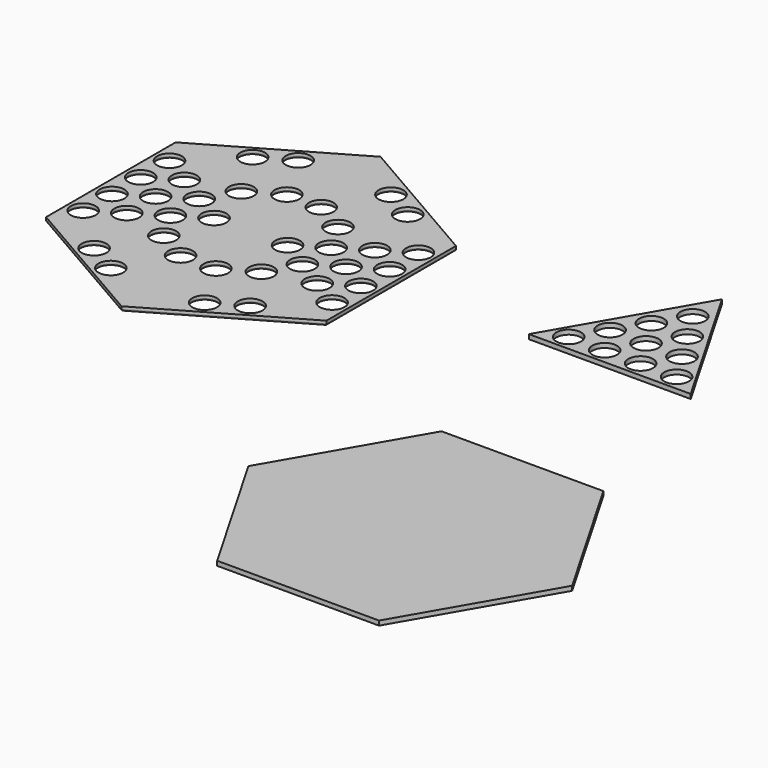
from build123d import *

# Parameters (mm, degrees)
F0_R        = 34.925
F1_DEPTH    = 12.7
F3_DEPTH    = 12.7
F4_T1_DEPTH = 482.6
F4_T3_DEPTH = 482.6
F4_T5_DEPTH = 482.6
F4_T7_DEPTH = 482.6
F4_T9_DEPTH = 482.6


# Not quite as in the source:
# - a fillet or chamfer that OpenCascade refuses, or shapes differently, is made with other operations: its cross-section is extruded or revolved along the edge and cut away or added


with BuildPart() as f1:
    # F0 (on Top) → F1 (new body)
    with BuildSketch(Plane.XY):
        Polygon((784.5862163544, 0), (1241.7862163544, 0), (1013.1862163544, 395.9468146102), align=None)
        with BuildLine():
            ThreePointArc((896.5008747508, 44.45), (870.615129901, 10.7150405169), (831.3299375236, 26.9875))
            ThreePointArc((831.3299375236, 26.9875), (852.5366196006, 78.1849594831), (896.5008747508, 44.45))
        make_face(mode=Mode.SUBTRACT)
        with Locations((963.1758747508, 44.45)):
            Circle(F0_R, mode=Mode.SUBTRACT)
        with Locations((1064.7758747508, 44.45)):
            Circle(F0_R, mode=Mode.SUBTRACT)
        with BuildLine():
            ThreePointArc((1201.3008747508, 44.45), (1200.0064823043, 35.0299224745), (1196.2192506657, 26.3080999065))
            ThreePointArc((1196.2192506657, 26.3080999065), (1132.7452671974, 53.8700775255), (1201.3008747508, 44.45))
        make_face(mode=Mode.SUBTRACT)
        with Locations((912.3758747508, 127)):
            Circle(F0_R, mode=Mode.SUBTRACT)
        with Locations((1013.9758747508, 127)):
            Circle(F0_R, mode=Mode.SUBTRACT)
        with BuildLine():
            ThreePointArc((963.1758747508, 174.625), (938.4801704179, 234.2457043329), (998.1008747508, 209.55))
            ThreePointArc((998.1008747508, 209.55), (987.8715790837, 184.8542956671), (963.1758747508, 174.625))
        make_face(mode=Mode.SUBTRACT)
        with Locations((1115.5758747508, 127)):
            Circle(F0_R, mode=Mode.SUBTRACT)
        with Locations((1064.7758747508, 209.55)):
            Circle(F0_R, mode=Mode.SUBTRACT)
        with BuildLine():
            ThreePointArc((1013.9758747508, 257.175), (989.2801704179, 316.7957043329), (1048.9008747508, 292.1))
            ThreePointArc((1048.9008747508, 292.1), (1038.6715790837, 267.4042956671), (1013.9758747508, 257.175))
        make_face(mode=Mode.SUBTRACT)
    extrude(amount=F1_DEPTH)


with BuildPart() as f1b:
    # F0 (on Top) → F1, piece 2 (new body)
    with BuildSketch(Plane.XY):
        Polygon((0, 0), (0, -457.2), (395.9468146102, -228.6), align=None)
        with Locations((132.4381810245, -329.4103416036)):
            Circle(F0_R, mode=Mode.SUBTRACT)
        with Locations((220.426362049, -278.6103416036)):
            Circle(F0_R, mode=Mode.SUBTRACT)
        with Locations((49.8881810245, -186.4295474388)):
            Circle(F0_R, mode=Mode.SUBTRACT)
        with Locations((137.876362049, -135.6295474388)):
            Circle(F0_R, mode=Mode.SUBTRACT)
        Polygon((-395.9468146102, -228.6), (0, -457.2), (0, 0), align=None)
        with Locations((-220.426362049, -278.6103416036)):
            Circle(F0_R, mode=Mode.SUBTRACT)
        with Locations((-132.4381810245, -329.4103416036)):
            Circle(F0_R, mode=Mode.SUBTRACT)
        with Locations((-49.8881810245, -186.4295474388)):
            Circle(F0_R, mode=Mode.SUBTRACT)
        with Locations((-137.876362049, -135.6295474388)):
            Circle(F0_R, mode=Mode.SUBTRACT)
        Polygon((-395.9468146102, 228.6), (-395.9468146102, -228.6), (0, 0), align=None)
        with Locations((-351.4968146102, -153.1896583964)):
            Circle(F0_R, mode=Mode.SUBTRACT)
        with Locations((-268.9468146102, -102.3896583964)):
            Circle(F0_R, mode=Mode.SUBTRACT)
        with Locations((-351.4968146102, -51.5896583964)):
            Circle(F0_R, mode=Mode.SUBTRACT)
        with Locations((-268.9468146102, -0.7896583964)):
            Circle(F0_R, mode=Mode.SUBTRACT)
        with Locations((-186.3968146102, -51.5896583964)):
            Circle(F0_R, mode=Mode.SUBTRACT)
        with Locations((-103.8468146102, -0.7896583964)):
            Circle(F0_R, mode=Mode.SUBTRACT)
        with Locations((-351.4968146102, 50.0103416036)):
            Circle(F0_R, mode=Mode.SUBTRACT)
        with Locations((-268.9468146102, 100.8103416036)):
            Circle(F0_R, mode=Mode.SUBTRACT)
        with Locations((-186.3968146102, 50.0103416036)):
            Circle(F0_R, mode=Mode.SUBTRACT)
        with Locations((-351.4968146102, 151.6103416036)):
            Circle(F0_R, mode=Mode.SUBTRACT)
        Polygon((0, 0), (395.9468146102, -228.6), (395.9468146102, 228.6), align=None)
        with Locations((351.4968146102, -153.1896583964)):
            Circle(F0_R, mode=Mode.SUBTRACT)
        with Locations((103.8468146102, -0.7896583964)):
            Circle(F0_R, mode=Mode.SUBTRACT)
        with Locations((186.3968146102, -51.5896583964)):
            Circle(F0_R, mode=Mode.SUBTRACT)
        with Locations((268.9468146102, -102.3896583964)):
            Circle(F0_R, mode=Mode.SUBTRACT)
        with Locations((268.9468146102, -0.7896583964)):
            Circle(F0_R, mode=Mode.SUBTRACT)
        with Locations((351.4968146102, -51.5896583964)):
            Circle(F0_R, mode=Mode.SUBTRACT)
        with Locations((186.3968146102, 50.0103416036)):
            Circle(F0_R, mode=Mode.SUBTRACT)
        with Locations((351.4968146102, 50.0103416036)):
            Circle(F0_R, mode=Mode.SUBTRACT)
        with Locations((268.9468146102, 100.8103416036)):
            Circle(F0_R, mode=Mode.SUBTRACT)
        with Locations((351.4968146102, 151.6103416036)):
            Circle(F0_R, mode=Mode.SUBTRACT)
        Polygon((0, 457.2), (0, 0), (395.9468146102, 228.6), align=None)
        with Locations((136.5086335857, 136.4192058352)):
            Circle(F0_R, mode=Mode.SUBTRACT)
        with Locations((48.5204525612, 187.2192058352)):
            Circle(F0_R, mode=Mode.SUBTRACT)
        with Locations((131.0704525612, 330.2)):
            Circle(F0_R, mode=Mode.SUBTRACT)
        with Locations((219.0586335857, 279.4)):
            Circle(F0_R, mode=Mode.SUBTRACT)
        Polygon((-395.9468146102, 228.6), (0, 0), (0, 457.2), align=None)
        with Locations((-136.5086335857, 136.4192058352)):
            Circle(F0_R, mode=Mode.SUBTRACT)
        with Locations((-48.5204525612, 187.2192058352)):
            Circle(F0_R, mode=Mode.SUBTRACT)
        with Locations((-219.0586335857, 279.4)):
            Circle(F0_R, mode=Mode.SUBTRACT)
        with Locations((-131.0704525612, 330.2)):
            Circle(F0_R, mode=Mode.SUBTRACT)
    extrude(amount=F1_DEPTH)

    # F4: fillet of radius 5.08 on 42 edges, made by hand

    # F4_s2 → F4_t1 (cut)
    with BuildSketch(Plane.XZ.offset(-241.3)):
        with BuildLine():
            ThreePointArc((-395.9468146102, 5.08), (-394.4589170587, 1.4878975516), (-390.8668146102, 0))
            Line((-390.8668146102, 0), (-395.9468146102, 0))
            Line((-395.9468146102, 0), (-395.9468146102, 5.08))
        make_face()
        with BuildLine():
            ThreePointArc((395.9468146102, 5.08), (394.4589170587, 1.4878975516), (390.8668146102, 0))
            Line((390.8668146102, 0), (395.9468146102, 0))
            Line((395.9468146102, 0), (395.9468146102, 5.08))
        make_face()
    extrude(amount=F4_T1_DEPTH, mode=Mode.SUBTRACT)

    # F4_s4 → F4_t3 (cut)
    with BuildSketch(Plane(origin=(-208.9719299332, 120.65, 0), x_dir=(0, 0, 1), z_dir=(0.8660254038, -0.5, 0))):
        with BuildLine():
            ThreePointArc((5.08, 395.9468146102), (1.4878975516, 394.4589170587), (0, 390.8668146102))
            Line((0, 390.8668146102), (0, 395.9468146102))
            Line((0, 395.9468146102), (5.08, 395.9468146102))
        make_face()
    extrude(amount=F4_T3_DEPTH, mode=Mode.SUBTRACT)

    # F4_s6 → F4_t5 (cut)
    with BuildSketch(Plane(origin=(-208.9719299332, -120.65, 0), x_dir=(0, 0, 1), z_dir=(0.8660254038, 0.5, 0))):
        with BuildLine():
            ThreePointArc((5.08, 395.9468146102), (1.4878975516, 394.4589170587), (0, 390.8668146102))
            Line((0, 390.8668146102), (0, 395.9468146102))
            Line((0, 395.9468146102), (5.08, 395.9468146102))
        make_face()
    extrude(amount=F4_T5_DEPTH, mode=Mode.SUBTRACT)

    # F4_s8 → F4_t7 (cut)
    with BuildSketch(Plane(origin=(208.9719299332, -120.65, 0), x_dir=(0, 0, 1), z_dir=(-0.8660254038, 0.5, 0))):
        with BuildLine():
            ThreePointArc((5.08, 395.9468146102), (1.4878975516, 394.4589170587), (0, 390.8668146102))
            Line((0, 390.8668146102), (0, 395.9468146102))
            Line((0, 395.9468146102), (5.08, 395.9468146102))
        make_face()
    extrude(amount=F4_T7_DEPTH, mode=Mode.SUBTRACT)

    # F4_s10 → F4_t9 (cut)
    with BuildSketch(Plane(origin=(208.9719299332, 120.65, 0), x_dir=(0, 0, 1), z_dir=(-0.8660254038, -0.5, 0))):
        with BuildLine():
            ThreePointArc((5.08, 395.9468146102), (1.4878975516, 394.4589170587), (0, 390.8668146102))
            Line((0, 390.8668146102), (0, 395.9468146102))
            Line((0, 395.9468146102), (5.08, 395.9468146102))
        make_face()
    extrude(amount=F4_T9_DEPTH, mode=Mode.SUBTRACT)

    # F4_s11 → F4_t12 (revolve, cut)
    with BuildSketch(Plane.XZ.offset(329.4103416036)):
        with BuildLine():
            ThreePointArc((167.3631810245, 5.08), (168.8510785761, 1.4878975516), (172.4431810245, 0))
            Line((172.4431810245, 0), (167.3631810245, 0))
            Line((167.3631810245, 0), (167.3631810245, 5.08))
        make_face()
    revolve(axis=Axis((132.4381810245, -329.4103416036, 0), (0, 0, 1)), mode=Mode.SUBTRACT)

    # F4_s13 → F4_t14 (revolve, cut)
    with BuildSketch(Plane.XZ.offset(278.6103416036)):
        with BuildLine():
            ThreePointArc((255.351362049, 5.08), (256.8392596006, 1.4878975516), (260.431362049, 0))
            Line((260.431362049, 0), (255.351362049, 0))
            Line((255.351362049, 0), (255.351362049, 5.08))
        make_face()
    revolve(axis=Axis((220.426362049, -278.6103416036, 0), (0, 0, 1)), mode=Mode.SUBTRACT)

    # F4_s15 → F4_t16 (revolve, cut)
    with BuildSketch(Plane.XZ.offset(186.4295474388)):
        with BuildLine():
            ThreePointArc((84.8131810245, 5.08), (86.3010785761, 1.4878975516), (89.8931810245, 0))
            Line((89.8931810245, 0), (84.8131810245, 0))
            Line((84.8131810245, 0), (84.8131810245, 5.08))
        make_face()
    revolve(axis=Axis((49.8881810245, -186.4295474388, 0), (0, 0, 1)), mode=Mode.SUBTRACT)

    # F4_s17 → F4_t18 (revolve, cut)
    with BuildSketch(Plane.XZ.offset(135.6295474388)):
        with BuildLine():
            ThreePointArc((172.801362049, 5.08), (174.2892596006, 1.4878975516), (177.881362049, 0))
            Line((177.881362049, 0), (172.801362049, 0))
            Line((172.801362049, 0), (172.801362049, 5.08))
        make_face()
    revolve(axis=Axis((137.876362049, -135.6295474388, 0), (0, 0, 1)), mode=Mode.SUBTRACT)

    # F4_s19 → F4_t20 (revolve, cut)
    with BuildSketch(Plane.XZ.offset(135.6295474388)):
        with BuildLine():
            ThreePointArc((-102.951362049, 5.08), (-101.4634644974, 1.4878975516), (-97.871362049, 0))
            Line((-97.871362049, 0), (-102.951362049, 0))
            Line((-102.951362049, 0), (-102.951362049, 5.08))
        make_face()
    revolve(axis=Axis((-137.876362049, -135.6295474388, 0), (0, 0, 1)), mode=Mode.SUBTRACT)

    # F4_s21 → F4_t22 (revolve, cut)
    with BuildSketch(Plane.XZ.offset(278.6103416036)):
        with BuildLine():
            ThreePointArc((-185.501362049, 5.08), (-184.0134644974, 1.4878975516), (-180.421362049, 0))
            Line((-180.421362049, 0), (-185.501362049, 0))
            Line((-185.501362049, 0), (-185.501362049, 5.08))
        make_face()
    revolve(axis=Axis((-220.426362049, -278.6103416036, 0), (0, 0, 1)), mode=Mode.SUBTRACT)

    # F4_s23 → F4_t24 (revolve, cut)
    with BuildSketch(Plane.XZ.offset(329.4103416036)):
        with BuildLine():
            ThreePointArc((-97.5131810245, 5.08), (-96.0252834729, 1.4878975516), (-92.4331810245, 0))
            Line((-92.4331810245, 0), (-97.5131810245, 0))
            Line((-97.5131810245, 0), (-97.5131810245, 5.08))
        make_face()
    revolve(axis=Axis((-132.4381810245, -329.4103416036, 0), (0, 0, 1)), mode=Mode.SUBTRACT)

    # F4_s25 → F4_t26 (revolve, cut)
    with BuildSketch(Plane.XZ.offset(186.4295474388)):
        with BuildLine():
            ThreePointArc((-14.9631810245, 5.08), (-13.4752834729, 1.4878975516), (-9.8831810245, 0))
            Line((-9.8831810245, 0), (-14.9631810245, 0))
            Line((-14.9631810245, 0), (-14.9631810245, 5.08))
        make_face()
    revolve(axis=Axis((-49.8881810245, -186.4295474388, 0), (0, 0, 1)), mode=Mode.SUBTRACT)

    # F4_s27 → F4_t28 (revolve, cut)
    with BuildSketch(Plane.XZ.offset(-151.6103416036)):
        with BuildLine():
            ThreePointArc((-316.5718146102, 5.08), (-315.0839170587, 1.4878975516), (-311.4918146102, 0))
            Line((-311.4918146102, 0), (-316.5718146102, 0))
            Line((-316.5718146102, 0), (-316.5718146102, 5.08))
        make_face()
    revolve(axis=Axis((-351.4968146102, 151.6103416036, 0), (0, 0, 1)), mode=Mode.SUBTRACT)

    # F4_s29 → F4_t30 (revolve, cut)
    with BuildSketch(Plane.XZ.offset(153.1896583964)):
        with BuildLine():
            ThreePointArc((-316.5718146102, 5.08), (-315.0839170587, 1.4878975516), (-311.4918146102, 0))
            Line((-311.4918146102, 0), (-316.5718146102, 0))
            Line((-316.5718146102, 0), (-316.5718146102, 5.08))
        make_face()
    revolve(axis=Axis((-351.4968146102, -153.1896583964, 0), (0, 0, 1)), mode=Mode.SUBTRACT)

    # F4_s31 → F4_t32 (revolve, cut)
    with BuildSketch(Plane.XZ.offset(102.3896583964)):
        with BuildLine():
            ThreePointArc((-234.0218146102, 5.08), (-232.5339170587, 1.4878975516), (-228.9418146102, 0))
            Line((-228.9418146102, 0), (-234.0218146102, 0))
            Line((-234.0218146102, 0), (-234.0218146102, 5.08))
        make_face()
    revolve(axis=Axis((-268.9468146102, -102.3896583964, 0), (0, 0, 1)), mode=Mode.SUBTRACT)

    # F4_s33 → F4_t34 (revolve, cut)
    with BuildSketch(Plane.XZ.offset(51.5896583964)):
        with BuildLine():
            ThreePointArc((-316.5718146102, 5.08), (-315.0839170587, 1.4878975516), (-311.4918146102, 0))
            Line((-311.4918146102, 0), (-316.5718146102, 0))
            Line((-316.5718146102, 0), (-316.5718146102, 5.08))
        make_face()
    revolve(axis=Axis((-351.4968146102, -51.5896583964, 0), (0, 0, 1)), mode=Mode.SUBTRACT)

    # F4_s35 → F4_t36 (revolve, cut)
    with BuildSketch(Plane.XZ.offset(0.7896583964)):
        with BuildLine():
            ThreePointArc((-234.0218146102, 5.08), (-232.5339170587, 1.4878975516), (-228.9418146102, 0))
            Line((-228.9418146102, 0), (-234.0218146102, 0))
            Line((-234.0218146102, 0), (-234.0218146102, 5.08))
        make_face()
    revolve(axis=Axis((-268.9468146102, -0.7896583964, 0), (0, 0, 1)), mode=Mode.SUBTRACT)

    # F4_s37 → F4_t38 (revolve, cut)
    with BuildSketch(Plane.XZ.offset(51.5896583964)):
        with BuildLine():
            ThreePointArc((-151.4718146102, 5.08), (-149.9839170587, 1.4878975516), (-146.3918146102, 0))
            Line((-146.3918146102, 0), (-151.4718146102, 0))
            Line((-151.4718146102, 0), (-151.4718146102, 5.08))
        make_face()
    revolve(axis=Axis((-186.3968146102, -51.5896583964, 0), (0, 0, 1)), mode=Mode.SUBTRACT)

    # F4_s39 → F4_t40 (revolve, cut)
    with BuildSketch(Plane.XZ.offset(0.7896583964)):
        with BuildLine():
            ThreePointArc((-68.9218146102, 5.08), (-67.4339170587, 1.4878975516), (-63.8418146102, 0))
            Line((-63.8418146102, 0), (-68.9218146102, 0))
            Line((-68.9218146102, 0), (-68.9218146102, 5.08))
        make_face()
    revolve(axis=Axis((-103.8468146102, -0.7896583964, 0), (0, 0, 1)), mode=Mode.SUBTRACT)

    # F4_s41 → F4_t42 (revolve, cut)
    with BuildSketch(Plane.XZ.offset(-50.0103416036)):
        with BuildLine():
            ThreePointArc((-316.5718146102, 5.08), (-315.0839170587, 1.4878975516), (-311.4918146102, 0))
            Line((-311.4918146102, 0), (-316.5718146102, 0))
            Line((-316.5718146102, 0), (-316.5718146102, 5.08))
        make_face()
    revolve(axis=Axis((-351.4968146102, 50.0103416036, 0), (0, 0, 1)), mode=Mode.SUBTRACT)

    # F4_s43 → F4_t44 (revolve, cut)
    with BuildSketch(Plane.XZ.offset(-100.8103416036)):
        with BuildLine():
            ThreePointArc((-234.0218146102, 5.08), (-232.5339170587, 1.4878975516), (-228.9418146102, 0))
            Line((-228.9418146102, 0), (-234.0218146102, 0))
            Line((-234.0218146102, 0), (-234.0218146102, 5.08))
        make_face()
    revolve(axis=Axis((-268.9468146102, 100.8103416036, 0), (0, 0, 1)), mode=Mode.SUBTRACT)

    # F4_s45 → F4_t46 (revolve, cut)
    with BuildSketch(Plane.XZ.offset(-50.0103416036)):
        with BuildLine():
            ThreePointArc((-151.4718146102, 5.08), (-149.9839170587, 1.4878975516), (-146.3918146102, 0))
            Line((-146.3918146102, 0), (-151.4718146102, 0))
            Line((-151.4718146102, 0), (-151.4718146102, 5.08))
        make_face()
    revolve(axis=Axis((-186.3968146102, 50.0103416036, 0), (0, 0, 1)), mode=Mode.SUBTRACT)

    # F4_s47 → F4_t48 (revolve, cut)
    with BuildSketch(Plane.XZ.offset(-151.6103416036)):
        with BuildLine():
            ThreePointArc((386.4218146102, 5.08), (387.9097121618, 1.4878975516), (391.5018146102, 0))
            Line((391.5018146102, 0), (386.4218146102, 0))
            Line((386.4218146102, 0), (386.4218146102, 5.08))
        make_face()
    revolve(axis=Axis((351.4968146102, 151.6103416036, 0), (0, 0, 1)), mode=Mode.SUBTRACT)

    # F4_s49 → F4_t50 (revolve, cut)
    with BuildSketch(Plane.XZ.offset(153.1896583964)):
        with BuildLine():
            ThreePointArc((386.4218146102, 5.08), (387.9097121618, 1.4878975516), (391.5018146102, 0))
            Line((391.5018146102, 0), (386.4218146102, 0))
            Line((386.4218146102, 0), (386.4218146102, 5.08))
        make_face()
    revolve(axis=Axis((351.4968146102, -153.1896583964, 0), (0, 0, 1)), mode=Mode.SUBTRACT)

    # F4_s51 → F4_t52 (revolve, cut)
    with BuildSketch(Plane.XZ.offset(0.7896583964)):
        with BuildLine():
            ThreePointArc((138.7718146102, 5.08), (140.2597121618, 1.4878975516), (143.8518146102, 0))
            Line((143.8518146102, 0), (138.7718146102, 0))
            Line((138.7718146102, 0), (138.7718146102, 5.08))
        make_face()
    revolve(axis=Axis((103.8468146102, -0.7896583964, 0), (0, 0, 1)), mode=Mode.SUBTRACT)

    # F4_s53 → F4_t54 (revolve, cut)
    with BuildSketch(Plane.XZ.offset(51.5896583964)):
        with BuildLine():
            ThreePointArc((221.3218146102, 5.08), (222.8097121618, 1.4878975516), (226.4018146102, 0))
            Line((226.4018146102, 0), (221.3218146102, 0))
            Line((221.3218146102, 0), (221.3218146102, 5.08))
        make_face()
    revolve(axis=Axis((186.3968146102, -51.5896583964, 0), (0, 0, 1)), mode=Mode.SUBTRACT)

    # F4_s55 → F4_t56 (revolve, cut)
    with BuildSketch(Plane.XZ.offset(102.3896583964)):
        with BuildLine():
            ThreePointArc((303.8718146102, 5.08), (305.3597121618, 1.4878975516), (308.9518146102, 0))
            Line((308.9518146102, 0), (303.8718146102, 0))
            Line((303.8718146102, 0), (303.8718146102, 5.08))
        make_face()
    revolve(axis=Axis((268.9468146102, -102.3896583964, 0), (0, 0, 1)), mode=Mode.SUBTRACT)

    # F4_s57 → F4_t58 (revolve, cut)
    with BuildSketch(Plane.XZ.offset(0.7896583964)):
        with BuildLine():
            ThreePointArc((303.8718146102, 5.08), (305.3597121618, 1.4878975516), (308.9518146102, 0))
            Line((308.9518146102, 0), (303.8718146102, 0))
            Line((303.8718146102, 0), (303.8718146102, 5.08))
        make_face()
    revolve(axis=Axis((268.9468146102, -0.7896583964, 0), (0, 0, 1)), mode=Mode.SUBTRACT)

    # F4_s59 → F4_t60 (revolve, cut)
    with BuildSketch(Plane.XZ.offset(51.5896583964)):
        with BuildLine():
            ThreePointArc((386.4218146102, 5.08), (387.9097121618, 1.4878975516), (391.5018146102, 0))
            Line((391.5018146102, 0), (386.4218146102, 0))
            Line((386.4218146102, 0), (386.4218146102, 5.08))
        make_face()
    revolve(axis=Axis((351.4968146102, -51.5896583964, 0), (0, 0, 1)), mode=Mode.SUBTRACT)

    # F4_s61 → F4_t62 (revolve, cut)
    with BuildSketch(Plane.XZ.offset(-50.0103416036)):
        with BuildLine():
            ThreePointArc((221.3218146102, 5.08), (222.8097121618, 1.4878975516), (226.4018146102, 0))
            Line((226.4018146102, 0), (221.3218146102, 0))
            Line((221.3218146102, 0), (221.3218146102, 5.08))
        make_face()
    revolve(axis=Axis((186.3968146102, 50.0103416036, 0), (0, 0, 1)), mode=Mode.SUBTRACT)

    # F4_s63 → F4_t64 (revolve, cut)
    with BuildSketch(Plane.XZ.offset(-50.0103416036)):
        with BuildLine():
            ThreePointArc((386.4218146102, 5.08), (387.9097121618, 1.4878975516), (391.5018146102, 0))
            Line((391.5018146102, 0), (386.4218146102, 0))
            Line((386.4218146102, 0), (386.4218146102, 5.08))
        make_face()
    revolve(axis=Axis((351.4968146102, 50.0103416036, 0), (0, 0, 1)), mode=Mode.SUBTRACT)

    # F4_s65 → F4_t66 (revolve, cut)
    with BuildSketch(Plane.XZ.offset(-100.8103416036)):
        with BuildLine():
            ThreePointArc((303.8718146102, 5.08), (305.3597121618, 1.4878975516), (308.9518146102, 0))
            Line((308.9518146102, 0), (303.8718146102, 0))
            Line((303.8718146102, 0), (303.8718146102, 5.08))
        make_face()
    revolve(axis=Axis((268.9468146102, 100.8103416036, 0), (0, 0, 1)), mode=Mode.SUBTRACT)

    # F4_s67 → F4_t68 (revolve, cut)
    with BuildSketch(Plane.XZ.offset(-279.4)):
        with BuildLine():
            ThreePointArc((253.9836335857, 5.08), (255.4715311373, 1.4878975516), (259.0636335857, 0))
            Line((259.0636335857, 0), (253.9836335857, 0))
            Line((253.9836335857, 0), (253.9836335857, 5.08))
        make_face()
    revolve(axis=Axis((219.0586335857, 279.4, 0), (0, 0, 1)), mode=Mode.SUBTRACT)

    # F4_s69 → F4_t70 (revolve, cut)
    with BuildSketch(Plane.XZ.offset(-136.4192058352)):
        with BuildLine():
            ThreePointArc((171.4336335857, 5.08), (172.9215311373, 1.4878975516), (176.5136335857, 0))
            Line((176.5136335857, 0), (171.4336335857, 0))
            Line((171.4336335857, 0), (171.4336335857, 5.08))
        make_face()
    revolve(axis=Axis((136.5086335857, 136.4192058352, 0), (0, 0, 1)), mode=Mode.SUBTRACT)

    # F4_s71 → F4_t72 (revolve, cut)
    with BuildSketch(Plane.XZ.offset(-187.2192058352)):
        with BuildLine():
            ThreePointArc((83.4454525612, 5.08), (84.9333501128, 1.4878975516), (88.5254525612, 0))
            Line((88.5254525612, 0), (83.4454525612, 0))
            Line((83.4454525612, 0), (83.4454525612, 5.08))
        make_face()
    revolve(axis=Axis((48.5204525612, 187.2192058352, 0), (0, 0, 1)), mode=Mode.SUBTRACT)

    # F4_s73 → F4_t74 (revolve, cut)
    with BuildSketch(Plane.XZ.offset(-330.2)):
        with BuildLine():
            ThreePointArc((165.9954525612, 5.08), (167.4833501128, 1.4878975516), (171.0754525612, 0))
            Line((171.0754525612, 0), (165.9954525612, 0))
            Line((165.9954525612, 0), (165.9954525612, 5.08))
        make_face()
    revolve(axis=Axis((131.0704525612, 330.2, 0), (0, 0, 1)), mode=Mode.SUBTRACT)

    # F4_s75 → F4_t76 (revolve, cut)
    with BuildSketch(Plane.XZ.offset(-330.2)):
        with BuildLine():
            ThreePointArc((-96.1454525612, 5.08), (-94.6575550097, 1.4878975516), (-91.0654525612, 0))
            Line((-91.0654525612, 0), (-96.1454525612, 0))
            Line((-96.1454525612, 0), (-96.1454525612, 5.08))
        make_face()
    revolve(axis=Axis((-131.0704525612, 330.2, 0), (0, 0, 1)), mode=Mode.SUBTRACT)

    # F4_s77 → F4_t78 (revolve, cut)
    with BuildSketch(Plane.XZ.offset(-279.4)):
        with BuildLine():
            ThreePointArc((-184.1336335857, 5.08), (-182.6457360342, 1.4878975516), (-179.0536335857, 0))
            Line((-179.0536335857, 0), (-184.1336335857, 0))
            Line((-184.1336335857, 0), (-184.1336335857, 5.08))
        make_face()
    revolve(axis=Axis((-219.0586335857, 279.4, 0), (0, 0, 1)), mode=Mode.SUBTRACT)

    # F4_s79 → F4_t80 (revolve, cut)
    with BuildSketch(Plane.XZ.offset(-136.4192058352)):
        with BuildLine():
            ThreePointArc((-101.5836335857, 5.08), (-100.0957360342, 1.4878975516), (-96.5036335857, 0))
            Line((-96.5036335857, 0), (-101.5836335857, 0))
            Line((-101.5836335857, 0), (-101.5836335857, 5.08))
        make_face()
    revolve(axis=Axis((-136.5086335857, 136.4192058352, 0), (0, 0, 1)), mode=Mode.SUBTRACT)

    # F4_s81 → F4_t82 (revolve, cut)
    with BuildSketch(Plane.XZ.offset(-187.2192058352)):
        with BuildLine():
            ThreePointArc((-13.5954525612, 5.08), (-12.1075550097, 1.4878975516), (-8.5154525612, 0))
            Line((-8.5154525612, 0), (-13.5954525612, 0))
            Line((-13.5954525612, 0), (-13.5954525612, 5.08))
        make_face()
    revolve(axis=Axis((-48.5204525612, 187.2192058352, 0), (0, 0, 1)), mode=Mode.SUBTRACT)


with BuildPart() as f3:
    # F2 (on Top) → F3 (new body)
    with BuildSketch(Plane.XY):
        Polygon((924.060369873, -1274.5785256164), (1381.260369873, -1274.5785256164), (1609.860369873, -878.6317110062), (1381.260369873, -482.6848963959), (924.060369873, -482.6848963959), (695.460369873, -878.6317110062), align=None)
    extrude(amount=F3_DEPTH)


solid = Compound([f1.part, f1b.part, f3.part])
